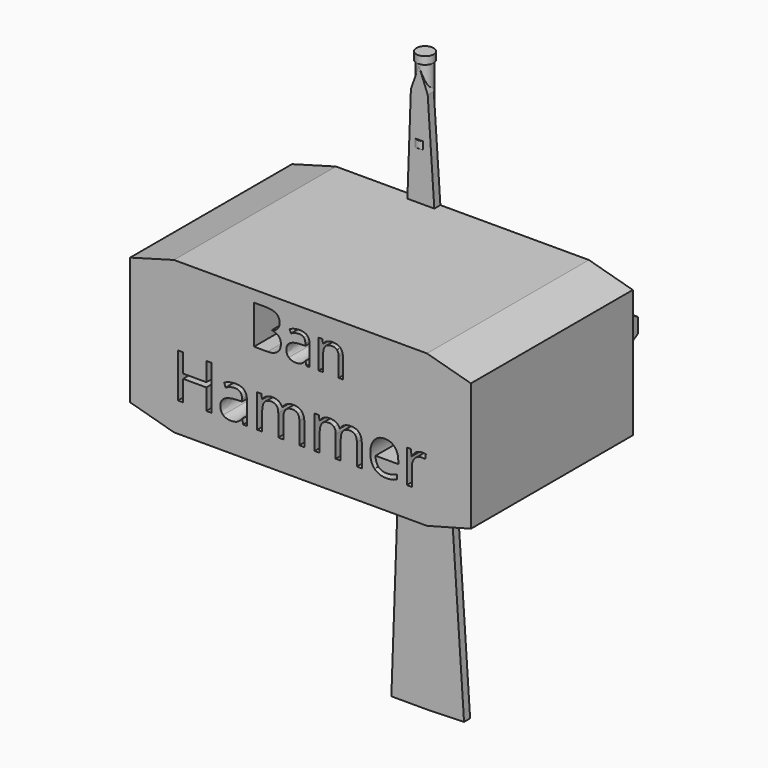
from build123d import *

# Parameters (mm, degrees)
F3_DEPTH = 80
F5_DEPTH = 3
F6_W     = 100
F6_H     = 60
F7_DEPTH = 80


# Not quite as in the source:
# - a feature names something its author has since deleted; it is built from what else it names


with BuildPart() as f1:
    # F0 (on Front) → F1 (revolve)
    with BuildSketch(Plane.XZ):
        Polygon((0, 71.4792597871), (-3, 71.4792597871), (-3.4, 71.4792597871), (-3.4, 68.4792597871), (-3.0011154904, 68.4792597871), (-3, 68.4792597871), (-3, 41.8595522642), (-3.4, 41.8595522642), (-3.4, 38.9757417142), (-3, 38.9757417142), (-3, 8.9757417142), (-3.4, 8.9757417142), (-3.4001515869, 5.9757417181), (-3.0001515869, 5.9757417181), (0, 5.9757417181), align=None)
    revolve(axis=Axis((0, 0, 38.7275007526), (0, 0, -1)))


with BuildPart() as f3:
    # F2 (on Right) → F3 (new body)
    with BuildSketch(Plane.YZ):
        Polygon((5.1675109757, 2.9581152655), (0.0219525206, 5.954253412), (-5.1455584551, 2.9961381465), (-5.1675109757, -2.9581152655), (-0.0219525206, -5.954253412), (5.1455584551, -2.9961381465), align=None)
    extrude(amount=F3_DEPTH)


with BuildPart() as f5:
    # F4 (on Front) → F5 (new body)
    with BuildSketch(Plane.XZ):
        Polygon((3.4626626875, 58.619774878), (0, 67.5975084305), (-3.1822064081, 58.5165781366), (-10.9075102955, -155.3643792868), (3.4626626875, -155.3643792868), (17.825905461, -154.9181410187), align=None)
    extrude(amount=F5_DEPTH)


with BuildPart() as f7:
    # F6 (on Front) → F7 (new body)
    with BuildSketch(Plane.XZ):
        Polygon((-35.2224066808, -40.1133835914), (-35.2224066808, 19.8866164086), (-52.5668375194, 15.0730191171), (-52.5668375194, -35.2997863), align=None)
        Polygon((82.1307391379, 15.1045321145), (64.7775933192, 19.8866164086), (64.7775933192, -40.1133835914), (82.1665007748, -35.4630182829), align=None)
        with Locations((14.7775933192, -10.1133835914)):
            Rectangle(F6_W, F6_H)
        Polygon((-20.4050052867, -11.0740224997), (-20.4050052867, -28.5098245367), (-22.4313591676, -28.5098245367), (-22.4313591676, -20.3051901792), (-31.616733539, -20.3051901792), (-31.616733539, -28.5098245367), (-33.6430874199, -28.5098245367), (-33.6430874199, -11.0740224997), (-31.616733539, -11.0740224997), (-31.616733539, -18.4925384025), (-22.4313591676, -18.4925384025), (-22.4313591676, -11.0740224997), align=None, mode=Mode.SUBTRACT)
        with BuildLine():
            Line((-6.4151496798, -28.5098245367), (-7.8843516462, -28.5098245367))
            Line((-7.8843516462, -28.5098245367), (-8.2774108735, -26.647563343))
            Line((-8.2774108735, -26.647563343), (-8.3728135986, -26.647563343))
            add(Edge.make_bspline(
                [(-8.3728135986, -26.647563343), (-9.3497375035, -27.8763504422), (-10.3209372449, -28.3132949231)],
                knots=[0, 0, 0, 1, 1, 1], degree=2))
            add(Edge.make_bspline(
                [(-10.3209372449, -28.3132949231), (-11.2921369863, -28.750239404), (-12.7498906257, -28.750239404)],
                knots=[0, 0, 0, 1, 1, 1], degree=2))
            add(Edge.make_bspline(
                [(-12.7498906257, -28.750239404), (-14.6922901084, -28.750239404), (-15.7951456105, -27.746602736)],
                knots=[0, 0, 0, 1, 1, 1], degree=2))
            add(Edge.make_bspline(
                [(-15.7951456105, -27.746602736), (-16.8980011125, -26.7429660681), (-16.8980011125, -24.8959693104)],
                knots=[0, 0, 0, 1, 1, 1], degree=2))
            add(Edge.make_bspline(
                [(-16.8980011125, -24.8959693104), (-16.8980011125, -20.9386642738), (-10.5670762756, -20.7478588236)],
                knots=[0, 0, 0, 1, 1, 1], degree=2))
            Line((-10.5670762756, -20.7478588236), (-8.3499169446, -20.6753527525))
            Line((-8.3499169446, -20.6753527525), (-8.3499169446, -19.8625215348))
            add(Edge.make_bspline(
                [(-8.3499169446, -19.8625215348), (-8.3499169446, -18.3246296064), (-9.0101038022, -17.5919366777)],
                knots=[0, 0, 0, 1, 1, 1], degree=2))
            add(Edge.make_bspline(
                [(-9.0101038022, -17.5919366777), (-9.6702906598, -16.859243749), (-11.1280442992, -16.859243749)],
                knots=[0, 0, 0, 1, 1, 1], degree=2))
            add(Edge.make_bspline(
                [(-11.1280442992, -16.859243749), (-12.7613389527, -16.859243749), (-14.8220378146, -17.8590643079)],
                knots=[0, 0, 0, 1, 1, 1], degree=2))
            Line((-14.8220378146, -17.8590643079), (-15.4326152551, -16.3440690335))
            add(Edge.make_bspline(
                [(-15.4326152551, -16.3440690335), (-14.4671396772, -15.8212621001), (-13.3165828127, -15.5236055978)],
                knots=[0, 0, 0, 1, 1, 1], degree=2))
            add(Edge.make_bspline(
                [(-13.3165828127, -15.5236055978), (-12.1660259481, -15.2259490955), (-11.005928811, -15.2259490955)],
                knots=[0, 0, 0, 1, 1, 1], degree=2))
            add(Edge.make_bspline(
                [(-11.005928811, -15.2259490955), (-8.6704701009, -15.2259490955), (-7.5428098904, -16.26202269)],
                knots=[0, 0, 0, 1, 1, 1], degree=2))
            add(Edge.make_bspline(
                [(-7.5428098904, -16.26202269), (-6.4151496798, -17.2980962844), (-6.4151496798, -19.5877616865)],
                knots=[0, 0, 0, 1, 1, 1], degree=2))
            Line((-6.4151496798, -19.5877616865), (-6.4151496798, -28.5098245367))
        make_face(mode=Mode.SUBTRACT)
        with BuildLine():
            Line((16.2983311091, -28.5098245367), (14.3215866453, -28.5098245367))
            Line((14.3215866453, -28.5098245367), (14.3215866453, -20.0075336769))
            add(Edge.make_bspline(
                [(14.3215866453, -20.0075336769), (14.3215866453, -18.4429289855), (13.6537675696, -17.6625346943)],
                knots=[0, 0, 0, 1, 1, 1], degree=2))
            add(Edge.make_bspline(
                [(13.6537675696, -17.6625346943), (12.985948494, -16.882140403), (11.5778042717, -16.882140403)],
                knots=[0, 0, 0, 1, 1, 1], degree=2))
            add(Edge.make_bspline(
                [(11.5778042717, -16.882140403), (9.730807514, -16.882140403), (8.8473782797, -17.943018706)],
                knots=[0, 0, 0, 1, 1, 1], degree=2))
            add(Edge.make_bspline(
                [(8.8473782797, -17.943018706), (7.9639490454, -19.003897009), (7.9639490454, -21.209608013)],
                knots=[0, 0, 0, 1, 1, 1], degree=2))
            Line((7.9639490454, -21.209608013), (7.9639490454, -28.5098245367))
            Line((7.9639490454, -28.5098245367), (5.9833884726, -28.5098245367))
            Line((5.9833884726, -28.5098245367), (5.9833884726, -20.0075336769))
            add(Edge.make_bspline(
                [(5.9833884726, -20.0075336769), (5.9833884726, -18.4429289855), (5.315569397, -17.6625346943)],
                knots=[0, 0, 0, 1, 1, 1], degree=2))
            add(Edge.make_bspline(
                [(5.315569397, -17.6625346943), (4.6477503214, -16.882140403), (3.2281577721, -16.882140403)],
                knots=[0, 0, 0, 1, 1, 1], degree=2))
            add(Edge.make_bspline(
                [(3.2281577721, -16.882140403), (1.3697126873, -16.882140403), (0.505363998, -17.9964442321)],
                knots=[0, 0, 0, 1, 1, 1], degree=2))
            add(Edge.make_bspline(
                [(0.505363998, -17.9964442321), (-0.3589846912, -19.1107480611), (-0.3589846912, -21.6522766574)],
                knots=[0, 0, 0, 1, 1, 1], degree=2))
            Line((-0.3589846912, -21.6522766574), (-0.3589846912, -28.5098245367))
            Line((-0.3589846912, -28.5098245367), (-2.3395452641, -28.5098245367))
            Line((-2.3395452641, -28.5098245367), (-2.3395452641, -15.4396511997))
            Line((-2.3395452641, -15.4396511997), (-0.7291472646, -15.4396511997))
            Line((-0.7291472646, -15.4396511997), (-0.4085941083, -17.2294063224))
            Line((-0.4085941083, -17.2294063224), (-0.3131913832, -17.2294063224))
            add(Edge.make_bspline(
                [(-0.3131913832, -17.2294063224), (0.2477766403, -16.2753790715), (1.2685857987, -15.737307702)],
                knots=[0, 0, 0, 1, 1, 1], degree=2))
            add(Edge.make_bspline(
                [(1.2685857987, -15.737307702), (2.2893949572, -15.1992363325), (3.5525270374, -15.1992363325)],
                knots=[0, 0, 0, 1, 1, 1], degree=2))
            add(Edge.make_bspline(
                [(3.5525270374, -15.1992363325), (6.6168625672, -15.1992363325), (7.559441491, -17.4202117725)],
                knots=[0, 0, 0, 1, 1, 1], degree=2))
            Line((7.559441491, -17.4202117725), (7.6548442161, -17.4202117725))
            add(Edge.make_bspline(
                [(7.6548442161, -17.4202117725), (8.2387088937, -16.3936784506), (9.3472885592, -15.7964573915)],
                knots=[0, 0, 0, 1, 1, 1], degree=2))
            add(Edge.make_bspline(
                [(9.3472885592, -15.7964573915), (10.4558682247, -15.1992363325), (11.875460774, -15.1992363325)],
                knots=[0, 0, 0, 1, 1, 1], degree=2))
            add(Edge.make_bspline(
                [(11.875460774, -15.1992363325), (14.0926201051, -15.1992363325), (15.1954756071, -16.33834487)],
                knots=[0, 0, 0, 1, 1, 1], degree=2))
            add(Edge.make_bspline(
                [(15.1954756071, -16.33834487), (16.2983311091, -17.4774534076), (16.2983311091, -19.9846370229)],
                knots=[0, 0, 0, 1, 1, 1], degree=2))
            Line((16.2983311091, -19.9846370229), (16.2983311091, -28.5098245367))
        make_face(mode=Mode.SUBTRACT)
        with BuildLine():
            Line((39.015628007, -28.5098245367), (37.0388835432, -28.5098245367))
            Line((37.0388835432, -28.5098245367), (37.0388835432, -20.0075336769))
            add(Edge.make_bspline(
                [(37.0388835432, -20.0075336769), (37.0388835432, -18.4429289855), (36.3710644676, -17.6625346943)],
                knots=[0, 0, 0, 1, 1, 1], degree=2))
            add(Edge.make_bspline(
                [(36.3710644676, -17.6625346943), (35.7032453919, -16.882140403), (34.2951011696, -16.882140403)],
                knots=[0, 0, 0, 1, 1, 1], degree=2))
            add(Edge.make_bspline(
                [(34.2951011696, -16.882140403), (32.4481044119, -16.882140403), (31.5646751776, -17.943018706)],
                knots=[0, 0, 0, 1, 1, 1], degree=2))
            add(Edge.make_bspline(
                [(31.5646751776, -17.943018706), (30.6812459433, -19.003897009), (30.6812459433, -21.209608013)],
                knots=[0, 0, 0, 1, 1, 1], degree=2))
            Line((30.6812459433, -21.209608013), (30.6812459433, -28.5098245367))
            Line((30.6812459433, -28.5098245367), (28.7006853705, -28.5098245367))
            Line((28.7006853705, -28.5098245367), (28.7006853705, -20.0075336769))
            add(Edge.make_bspline(
                [(28.7006853705, -20.0075336769), (28.7006853705, -18.4429289855), (28.0328662949, -17.6625346943)],
                knots=[0, 0, 0, 1, 1, 1], degree=2))
            add(Edge.make_bspline(
                [(28.0328662949, -17.6625346943), (27.3650472193, -16.882140403), (25.94545467, -16.882140403)],
                knots=[0, 0, 0, 1, 1, 1], degree=2))
            add(Edge.make_bspline(
                [(25.94545467, -16.882140403), (24.0870095852, -16.882140403), (23.222660896, -17.9964442321)],
                knots=[0, 0, 0, 1, 1, 1], degree=2))
            add(Edge.make_bspline(
                [(23.222660896, -17.9964442321), (22.3583122067, -19.1107480611), (22.3583122067, -21.6522766574)],
                knots=[0, 0, 0, 1, 1, 1], degree=2))
            Line((22.3583122067, -21.6522766574), (22.3583122067, -28.5098245367))
            Line((22.3583122067, -28.5098245367), (20.3777516338, -28.5098245367))
            Line((20.3777516338, -28.5098245367), (20.3777516338, -15.4396511997))
            Line((20.3777516338, -15.4396511997), (21.9881496333, -15.4396511997))
            Line((21.9881496333, -15.4396511997), (22.3087027896, -17.2294063224))
            Line((22.3087027896, -17.2294063224), (22.4041055147, -17.2294063224))
            add(Edge.make_bspline(
                [(22.4041055147, -17.2294063224), (22.9650735382, -16.2753790715), (23.9858826967, -15.737307702)],
                knots=[0, 0, 0, 1, 1, 1], degree=2))
            add(Edge.make_bspline(
                [(23.9858826967, -15.737307702), (25.0066918551, -15.1992363325), (26.2698239353, -15.1992363325)],
                knots=[0, 0, 0, 1, 1, 1], degree=2))
            add(Edge.make_bspline(
                [(26.2698239353, -15.1992363325), (29.3341594651, -15.1992363325), (30.2767383889, -17.4202117725)],
                knots=[0, 0, 0, 1, 1, 1], degree=2))
            Line((30.2767383889, -17.4202117725), (30.372141114, -17.4202117725))
            add(Edge.make_bspline(
                [(30.372141114, -17.4202117725), (30.9560057916, -16.3936784506), (32.0645854571, -15.7964573915)],
                knots=[0, 0, 0, 1, 1, 1], degree=2))
            add(Edge.make_bspline(
                [(32.0645854571, -15.7964573915), (33.1731651226, -15.1992363325), (34.5927576719, -15.1992363325)],
                knots=[0, 0, 0, 1, 1, 1], degree=2))
            add(Edge.make_bspline(
                [(34.5927576719, -15.1992363325), (36.809917003, -15.1992363325), (37.912772505, -16.33834487)],
                knots=[0, 0, 0, 1, 1, 1], degree=2))
            add(Edge.make_bspline(
                [(37.912772505, -16.33834487), (39.015628007, -17.4774534076), (39.015628007, -19.9846370229)],
                knots=[0, 0, 0, 1, 1, 1], degree=2))
            Line((39.015628007, -19.9846370229), (39.015628007, -28.5098245367))
        make_face(mode=Mode.SUBTRACT)
        with BuildLine():
            add(Edge.make_bspline(
                [(50.8760947899, -28.5518017358), (49.941148084, -28.750239404), (48.6169582598, -28.750239404)],
                knots=[0, 0, 0, 1, 1, 1], degree=2))
            add(Edge.make_bspline(
                [(48.6169582598, -28.750239404), (45.7205315262, -28.750239404), (44.0433516191, -26.9833809353)],
                knots=[0, 0, 0, 1, 1, 1], degree=2))
            add(Edge.make_bspline(
                [(44.0433516191, -26.9833809353), (42.3661717121, -25.2165224667), (42.3661717121, -22.0834969748)],
                knots=[0, 0, 0, 1, 1, 1], degree=2))
            add(Edge.make_bspline(
                [(42.3661717121, -22.0834969748), (42.3661717121, -18.9199426109), (43.9231441855, -17.0595894717)],
                knots=[0, 0, 0, 1, 1, 1], degree=2))
            add(Edge.make_bspline(
                [(43.9231441855, -17.0595894717), (45.4801166589, -15.1992363325), (48.1055996534, -15.1992363325)],
                knots=[0, 0, 0, 1, 1, 1], degree=2))
            add(Edge.make_bspline(
                [(48.1055996534, -15.1992363325), (50.5593577426, -15.1992363325), (51.9903986189, -16.8153584955)],
                knots=[0, 0, 0, 1, 1, 1], degree=2))
            add(Edge.make_bspline(
                [(51.9903986189, -16.8153584955), (53.4214394952, -18.4314806585), (53.4214394952, -21.0798603069)],
                knots=[0, 0, 0, 1, 1, 1], degree=2))
            Line((53.4214394952, -21.0798603069), (53.4214394952, -22.3315440601))
            Line((53.4214394952, -22.3315440601), (44.419238356, -22.3315440601))
            add(Edge.make_bspline(
                [(44.419238356, -22.3315440601), (44.4802961, -24.6326577892), (45.583151602, -25.8251918528)],
                knots=[0, 0, 0, 1, 1, 1], degree=2))
            add(Edge.make_bspline(
                [(45.583151602, -25.8251918528), (46.686007104, -27.0177259164), (48.6894643309, -27.0177259164)],
                knots=[0, 0, 0, 1, 1, 1], degree=2))
            add(Edge.make_bspline(
                [(48.6894643309, -27.0177259164), (50.7997726098, -27.0177259164), (52.8604714717, -26.1362047366)],
                knots=[0, 0, 0, 1, 1, 1], degree=2))
            Line((52.8604714717, -26.1362047366), (52.8604714717, -27.9030632052))
            add(Edge.make_bspline(
                [(52.8604714717, -27.9030632052), (51.8110414958, -28.3533640676), (50.8760947899, -28.5518017358)],
                knots=[0, 0, 0, 1, 1, 1], degree=2))
        make_face(mode=Mode.SUBTRACT)
        with BuildLine():
            add(Edge.make_bspline(
                [(60.5079539148, -15.8918601166), (61.5344872367, -15.1992363325), (62.7632743358, -15.1992363325)],
                knots=[0, 0, 0, 1, 1, 1], degree=2))
            add(Edge.make_bspline(
                [(62.7632743358, -15.1992363325), (63.6333471886, -15.1992363325), (64.3240629183, -15.3442484746)],
                knots=[0, 0, 0, 1, 1, 1], degree=2))
            Line((64.3240629183, -15.3442484746), (64.04930307, -17.1797969053))
            add(Edge.make_bspline(
                [(64.04930307, -17.1797969053), (63.2402879613, -17.0004397821), (62.6182621937, -17.0004397821)],
                knots=[0, 0, 0, 1, 1, 1], degree=2))
            add(Edge.make_bspline(
                [(62.6182621937, -17.0004397821), (61.0307608482, -17.0004397821), (59.9050086922, -18.2883765708)],
                knots=[0, 0, 0, 1, 1, 1], degree=2))
            add(Edge.make_bspline(
                [(59.9050086922, -18.2883765708), (58.7792565362, -19.5763133595), (58.7792565362, -21.4958161883)],
                knots=[0, 0, 0, 1, 1, 1], degree=2))
            Line((58.7792565362, -21.4958161883), (58.7792565362, -28.5098245367))
            Line((58.7792565362, -28.5098245367), (56.7986959634, -28.5098245367))
            Line((56.7986959634, -28.5098245367), (56.7986959634, -15.4396511997))
            Line((56.7986959634, -15.4396511997), (58.4319906169, -15.4396511997))
            Line((58.4319906169, -15.4396511997), (58.6609571571, -17.8590643079))
            Line((58.6609571571, -17.8590643079), (58.7563598822, -17.8590643079))
            add(Edge.make_bspline(
                [(58.7563598822, -17.8590643079), (59.4814205928, -16.5844839008), (60.5079539148, -15.8918601166)],
                knots=[0, 0, 0, 1, 1, 1], degree=2))
        make_face(mode=Mode.SUBTRACT)
        with BuildLine():
            Line((-3.5971520984, 0), (-3.5971520984, 15.3209723352))
            Line((-3.5971520984, 15.3209723352), (0.7318860466, 15.3209723352))
            add(Edge.make_bspline(
                [(0.7318860466, 15.3209723352), (3.7799849419, 15.3209723352), (5.1430786723, 14.4088899374)],
                knots=[0, 0, 0, 1, 1, 1], degree=2))
            add(Edge.make_bspline(
                [(5.1430786723, 14.4088899374), (6.5061724027, 13.4968075397), (6.5061724027, 11.5284532476)],
                knots=[0, 0, 0, 1, 1, 1], degree=2))
            add(Edge.make_bspline(
                [(6.5061724027, 11.5284532476), (6.5061724027, 10.1636828951), (5.746662612, 9.2784264503)],
                knots=[0, 0, 0, 1, 1, 1], degree=2))
            add(Edge.make_bspline(
                [(5.746662612, 9.2784264503), (4.9871528212, 8.3931700054), (3.5284916337, 8.1316169649)],
                knots=[0, 0, 0, 1, 1, 1], degree=2))
            Line((3.5284916337, 8.1316169649), (3.5284916337, 8.0276663975))
            add(Edge.make_bspline(
                [(3.5284916337, 8.0276663975), (7.0192187514, 7.4307889461), (7.0192187514, 4.359217342)],
                knots=[0, 0, 0, 1, 1, 1], degree=2))
            add(Edge.make_bspline(
                [(7.0192187514, 4.359217342), (7.0192187514, 2.3070319472), (5.6309756902, 1.1535159736)],
                knots=[0, 0, 0, 1, 1, 1], degree=2))
            add(Edge.make_bspline(
                [(5.6309756902, 1.1535159736), (4.242732629, 0), (1.7479190117, 0)],
                knots=[0, 0, 0, 1, 1, 1], degree=2))
            Line((1.7479190117, 0), (-3.5971520984, 0))
        make_face(mode=Mode.SUBTRACT)
        with BuildLine():
            Line((18.4001292582, 0), (17.1091302762, 0))
            Line((17.1091302762, 0), (16.7637461329, 1.6363831253))
            Line((16.7637461329, 1.6363831253), (16.6799150302, 1.6363831253))
            add(Edge.make_bspline(
                [(16.6799150302, 1.6363831253), (15.8214845382, 0.5566385221), (14.9680839124, 0.1726920716)],
                knots=[0, 0, 0, 1, 1, 1], degree=2))
            add(Edge.make_bspline(
                [(14.9680839124, 0.1726920716), (14.1146832866, -0.2112543789), (12.8337440369, -0.2112543789)],
                knots=[0, 0, 0, 1, 1, 1], degree=2))
            add(Edge.make_bspline(
                [(12.8337440369, -0.2112543789), (11.1269427853, -0.2112543789), (10.1578552377, 0.6706488218)],
                knots=[0, 0, 0, 1, 1, 1], degree=2))
            add(Edge.make_bspline(
                [(10.1578552377, 0.6706488218), (9.1887676901, 1.5525520226), (9.1887676901, 3.1755221715)],
                knots=[0, 0, 0, 1, 1, 1], degree=2))
            add(Edge.make_bspline(
                [(9.1887676901, 3.1755221715), (9.1887676901, 6.6528363127), (14.7517996674, 6.8204985182)],
                knots=[0, 0, 0, 1, 1, 1], degree=2))
            Line((14.7517996674, 6.8204985182), (16.7000344948, 6.8842101563))
            Line((16.7000344948, 6.8842101563), (16.7000344948, 7.5984511516))
            add(Edge.make_bspline(
                [(16.7000344948, 7.5984511516), (16.7000344948, 8.9498085276), (16.1199232639, 9.5936313966)],
                knots=[0, 0, 0, 1, 1, 1], degree=2))
            add(Edge.make_bspline(
                [(16.1199232639, 9.5936313966), (15.539812033, 10.2374542655), (14.2588727833, 10.2374542655)],
                knots=[0, 0, 0, 1, 1, 1], degree=2))
            add(Edge.make_bspline(
                [(14.2588727833, 10.2374542655), (12.8236843045, 10.2374542655), (11.0129324856, 9.3589043089)],
                knots=[0, 0, 0, 1, 1, 1], degree=2))
            Line((11.0129324856, 9.3589043089), (10.4764134281, 10.6901422203))
            add(Edge.make_bspline(
                [(10.4764134281, 10.6901422203), (11.3247841877, 11.1495366632), (12.3357872867, 11.4110897038)],
                knots=[0, 0, 0, 1, 1, 1], degree=2))
            add(Edge.make_bspline(
                [(12.3357872867, 11.4110897038), (13.3467903856, 11.6726427443), (14.3661765948, 11.6726427443)],
                knots=[0, 0, 0, 1, 1, 1], degree=2))
            add(Edge.make_bspline(
                [(14.3661765948, 11.6726427443), (16.4183619897, 11.6726427443), (17.4092456239, 10.7622369686)],
                knots=[0, 0, 0, 1, 1, 1], degree=2))
            add(Edge.make_bspline(
                [(17.4092456239, 10.7622369686), (18.4001292582, 9.851831193), (18.4001292582, 7.8398847274)],
                knots=[0, 0, 0, 1, 1, 1], degree=2))
            Line((18.4001292582, 7.8398847274), (18.4001292582, 0))
        make_face(mode=Mode.SUBTRACT)
        with BuildLine():
            Line((31.5817318517, 0), (29.841398159, 0))
            Line((29.841398159, 0), (29.841398159, 7.4307889461))
            add(Edge.make_bspline(
                [(29.841398159, 7.4307889461), (29.841398159, 8.8324449838), (29.2026051562, 9.5248898923)],
                knots=[0, 0, 0, 1, 1, 1], degree=2))
            add(Edge.make_bspline(
                [(29.2026051562, 9.5248898923), (28.5638121534, 10.2173348009), (27.1990418009, 10.2173348009)],
                knots=[0, 0, 0, 1, 1, 1], degree=2))
            add(Edge.make_bspline(
                [(27.1990418009, 10.2173348009), (25.3983497142, 10.2173348009), (24.5600386869, 9.2432173871)],
                knots=[0, 0, 0, 1, 1, 1], degree=2))
            add(Edge.make_bspline(
                [(24.5600386869, 9.2432173871), (23.7217276596, 8.2690999734), (23.7217276596, 6.0257796643)],
                knots=[0, 0, 0, 1, 1, 1], degree=2))
            Line((23.7217276596, 6.0257796643), (23.7217276596, 0))
            Line((23.7217276596, 0), (21.9813939669, 0))
            Line((21.9813939669, 0), (21.9813939669, 11.4848610742))
            Line((21.9813939669, 11.4848610742), (23.396462981, 11.4848610742))
            Line((23.396462981, 11.4848610742), (23.6781354862, 9.9121895869))
            Line((23.6781354862, 9.9121895869), (23.7619665889, 9.9121895869))
            add(Edge.make_bspline(
                [(23.7619665889, 9.9121895869), (24.2984856464, 10.7605603466), (25.2625433278, 11.2283378998)],
                knots=[0, 0, 0, 1, 1, 1], degree=2))
            add(Edge.make_bspline(
                [(25.2625433278, 11.2283378998), (26.2266010092, 11.6961154531), (27.4102961798, 11.6961154531)],
                knots=[0, 0, 0, 1, 1, 1], degree=2))
            add(Edge.make_bspline(
                [(27.4102961798, 11.6961154531), (29.4859542834, 11.6961154531), (30.5338430675, 10.6951720864)],
                knots=[0, 0, 0, 1, 1, 1], degree=2))
            add(Edge.make_bspline(
                [(30.5338430675, 10.6951720864), (31.5817318517, 9.6942287198), (31.5817318517, 7.4911473401)],
                knots=[0, 0, 0, 1, 1, 1], degree=2))
            Line((31.5817318517, 7.4911473401), (31.5817318517, 0))
        make_face(mode=Mode.SUBTRACT)
    extrude(amount=F7_DEPTH)


solid = Compound([f1.part, f3.part, f5.part, f7.part])
